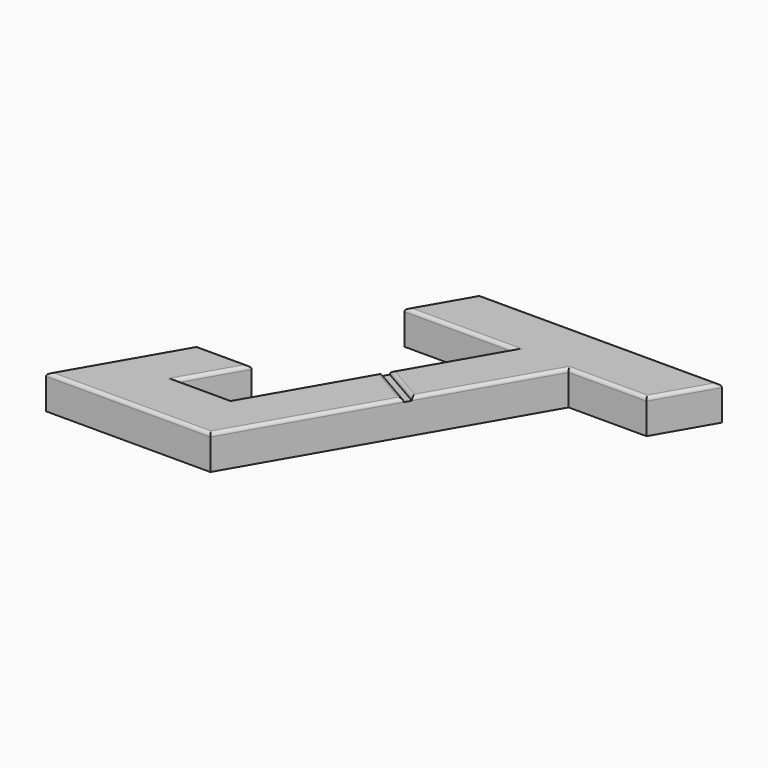
from build123d import *

# Parameters (mm, degrees)
F1_DEPTH = 5
F4_W     = 1
F4_H     = 5.3799478337
F5_DEPTH = 100
F6_T     = -0.75
F7_R     = 0.49999
F9_DEPTH = 4.25


# Not quite as in the source:
# - a fillet or chamfer is up to 0.001 mm smaller than in the source, because OpenCascade refuses the exact size


with BuildPart() as f1:
    # F0 (on Top) → F1 (new body)
    with BuildSketch(Plane.XY):
        Polygon((-15.3811978465, 38), (-20, 30), (-4, 30), (-21.3205080757, 0), (-29.3205080757, 0), (-24.7017059222, 8), (-32.7017059222, 8), (-41.9393102292, -8), (-17.9393102292, -8), (4, 30), (15.3811978465, 30), (20, 38), align=None)
    extrude(amount=F1_DEPTH)

    # F4 (on offset) → F5 (cut)
    with BuildSketch(Plane(origin=(11.6602540378, -6.7320508076, 0), x_dir=(0.5, 0.8660254038, 0), z_dir=(0.8660254038, -0.5, 0))):
        with Locations((8.2942286341, 7.1899739169)):
            Rectangle(F4_W, F4_H)
    extrude(amount=-F5_DEPTH, mode=Mode.SUBTRACT)

    # F6
    f6_openings = [f1.faces().sort_by_distance(p)[0] for p in [
        (2.309401, 37.228477, 0),
    ]]
    offset(amount=F6_T, openings=f6_openings, kind=Kind.INTERSECTION)

    # F7 (radius 0.5 in the source; OpenCascade refuses exactly that, so slightly less here)
    f7_edges = [f1.edges().sort_by_distance(p)[0] for p in [
        (-0.796633, 21.691987, 5),
        (9.690599, 30, 5),
        (17.690599, 34, 5),
        (2.309401, 38, 5),
        (-17.690599, 34, 5),
        (-12, 30, 5),
        (-7.796633, 23.424038, 5),
        (-8.593267, 15.116025, 5),
        (-16.706887, 7.991025, 5),
        (-25.320508, 0, 5),
        (-27.011107, 4, 5),
        (-28.701706, 8, 5),
        (-37.320508, 0, 5),
        (-29.93931, -8, 5),
        (-12.016288, 2.258975, 5),
        (-9.093267, 14.25, 5),
    ]]
    fillet(f7_edges, radius=F7_R)

    # F8 (on face) → F9 (join, through all)
    with BuildSketch(Plane(origin=(0, 0, 4.25), x_dir=(1, 0, 0), z_dir=(0, 0, -1))):
        Polygon((-10.5823786219, -30.75), (-12.9481851446, -37.25), (-10.9481851446, -37.25), (-8.5823786219, -30.75), align=None)
        Polygon((10.9481851446, -30.75), (8.5823786219, -37.25), (10.5823786219, -37.25), (12.9481851446, -30.75), align=None)
    extrude(amount=F9_DEPTH)


solid = f1.part
